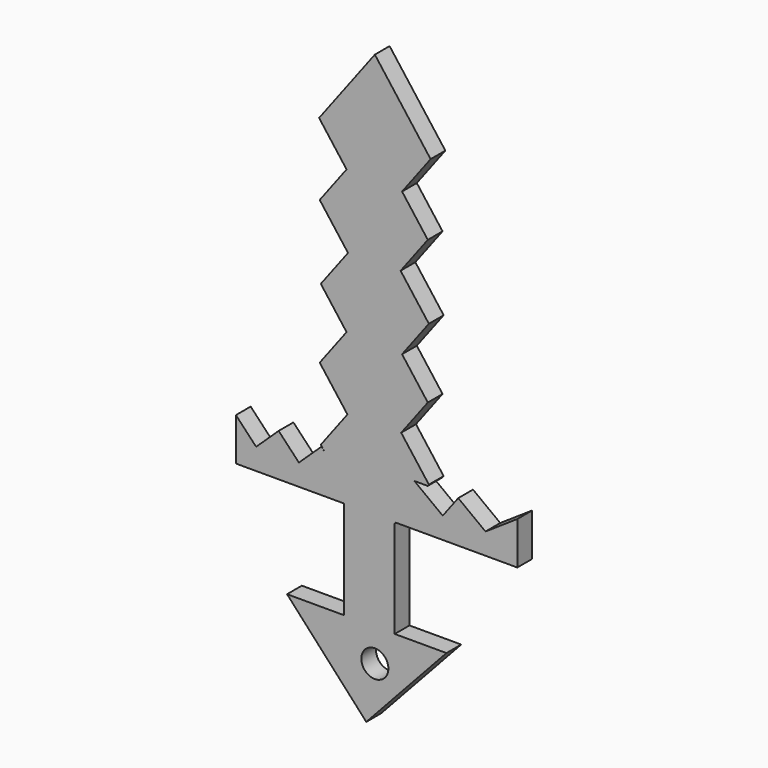
from build123d import *

# Parameters (mm, degrees)
F0_R     = 3.7313011015
F1_DEPTH = 5.08


# Not quite as in the source:
# - a feature names something its author has since deleted; it is built from what else it names


with BuildPart() as f1:
    # F0 (on Front) → F1 (new body)
    with BuildSketch(Plane.XZ):
        Polygon((-0.2968451337, 20.2413384518), (7.4894401646, 9.9239995871), (14.8768772094, 19.7128383483), (7.0905919112, 30.0301772131), (0, 39.4256766967), (-7.3874370448, 29.6368379354), (-14.8768772094, 19.7128383483), (-7.7862852982, 10.3173388647), align=None)
        Polygon((14.5800320757, 0.5285001035), (7.4894401646, 9.9239995871), (-0.2968451337, 20.2413384518), (-7.7862852982, 10.3173388647), (-15.1737223431, 0.5285001035), (-7.5532907703, -9.5690716936), (0, 0.4395341352), (7.2564456366, -9.175732416), align=None)
        Polygon((0, 39.4256766967), (7.0905919112, 30.0301772131), (14.5800320757, 39.9541768002), (7.4894401646, 49.3496762838), (-0.2968451337, 59.6670151485), (-7.7862852982, 49.7430155614), (-15.1737223431, 39.9541768002), (-7.3874370448, 29.6368379354), align=None)
        Polygon((14.8768772094, -19.2733042131), (7.2564456366, -9.175732416), (0, 0.4395341352), (-7.5532907703, -9.5690716936), (-14.8768772094, -19.2733042131), (-14.5568754898, -19.6973274863), (10.9024396727, -19.6973274863), (14.5568754898, -19.6973274863), align=None)
        Polygon((-0.2968451337, 59.6670151485), (7.4894401646, 49.3496762838), (15.3495463603, 59.7648326808), (0, 80.103988665), (-15.3495463602, 59.7648326808), (-7.7862852982, 49.7430155614), align=None)
        Polygon((6.4679318367, -25.5733413094), (10.9024396727, -19.6973274863), (-14.5568754898, -19.6973274863), (-13.9719483627, -20.4723943058), (-9.1415820241, -25.5733413094), (-1.0331695214, -19.9124130418), align=None)
        Polygon((18.6885435032, -25.5733413094), (10.9024396727, -19.6973274863), (6.4679318367, -25.5733413094), (-1.0331695214, -19.9124130418), (-9.1415820241, -25.5733413094), (-13.9719483627, -20.4723943058), (-14.7059016213, -19.6973274863), (-20.9110697187, -25.5733413094), (-26.4753893159, -19.6973274863), (-32.6805574134, -25.5733413094), (-38.2448770106, -19.6973274863), (-38.2448770106, -31.4493551324), (-8.4425376974, -31.4493551324), (5.4781014785, -31.4493551324), (5.6878598178, -31.4493551324), (39.2251229894, -31.4493551324), (39.2251229894, -19.6973274863), (30.4618320136, -25.5733413094), (22.9607306555, -19.9124130418), align=None)
        Polygon((5.4781014785, -31.7272986938), (5.6878598178, -31.4493551324), (5.4781014785, -31.4493551324), align=None)
        Polygon((5.4781014785, -58.5252254202), (5.4781014785, -31.7272986938), (5.4781014785, -31.4493551324), (-8.4425376974, -31.4493551324), (-8.4425376974, -58.5252254202), align=None)
        Polygon((19.711822737, -58.5252254202), (5.4781014785, -58.5252254202), (-8.4425376974, -58.5252254202), (-24.1670380346, -58.5252254202), (-2.355908975, -82.3924914002), align=None)
        with Locations((0, -67.5043612719)):
            Circle(F0_R, mode=Mode.SUBTRACT)
    extrude(amount=F1_DEPTH)


solid = f1.part
